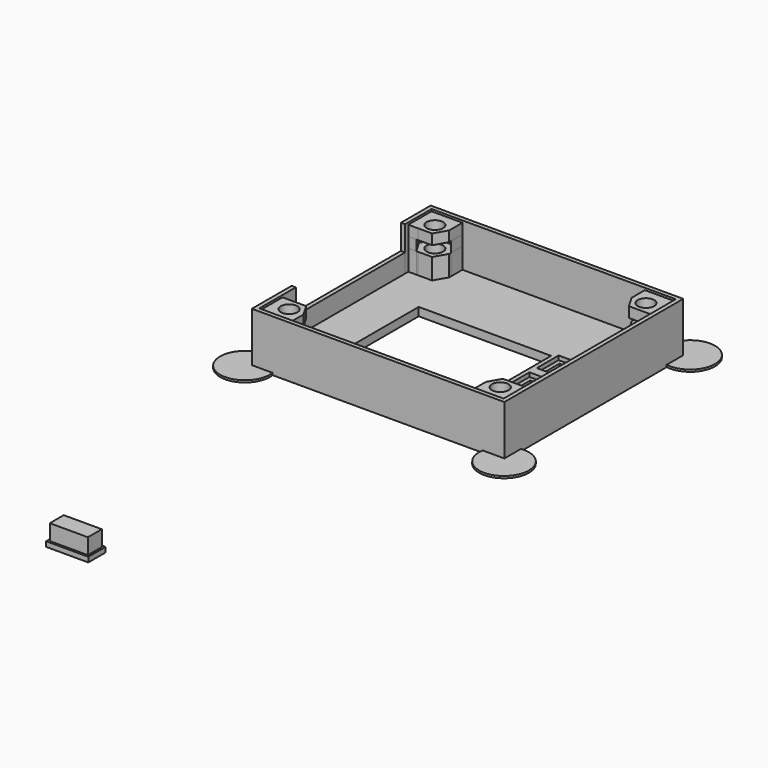
from build123d import *

# Parameters (mm, degrees)
F0_R      = 2
F1_DEPTH  = 7
F2_DEPTH  = 7
F3_DEPTH  = 2.5
F4_START  = 2.5
F1_FACE_R = 2
F4_DEPTH  = 2.5
F0_W      = 32
F0_H      = 23
F0_W_2    = 11.6
F0_H_2    = 6.6
F5_DEPTH  = 2
F0_W_3    = 9.6
F0_H_3    = 4.6
F6_DEPTH  = 1
F7_DEPTH  = 12.5
F0_W_4    = 1
F0_H_4    = 33
F8_DEPTH  = 6.5
F0_W_5    = 10.2
F0_H_5    = 5.2
F0_W_6    = 9.2
F0_H_6    = 4.2
F9_DEPTH  = 1.2
F10_DEPTH = 5
F11_DEPTH = 0.5


with BuildPart() as f1:
    # F0 (on Top) → F1 (new body)
    with BuildSketch(Plane.XY):
        Polygon((56.2425711751, 29.4110085815), (56.2425711751, 36.414245103), (54.3157895307, 36.414245103), (56.0530762776, 33.4181404888), (54.1540001392, 30.1145803152), (50.3434950368, 30.1074484079), (48.7784756274, 32.8064627658), (48.7784756274, 29.4110085815), (52.2425711751, 29.4110085815), align=None)
        Polygon((56.0530762776, 33.4181404888), (54.3157895307, 36.414245103), (53.9690040281, 36.414245103), (50.5049084804, 36.4077615509), (48.7784756274, 33.4045250294), (48.7784756274, 32.8064627658), (50.3434950368, 30.1074484079), (54.1540001392, 30.1145803152), align=None)
        with Locations((52.2425711751, 33.4110085815)):
            Circle(F0_R, mode=Mode.SUBTRACT)
    extrude(amount=F1_DEPTH)


with BuildPart() as f1b:
    # F0 (on Top) → F1, piece 2 (new body)
    with BuildSketch(Plane.XY):
        Polygon((-0.8411283625, 36.4077615509), (-2.7574288249, 36.4077615509), (-2.7574288249, 29.4110085815), (4.7066667228, 29.4110085815), (4.7066667228, 32.8155396842), (3.1540001392, 30.1145803152), (-0.6565049632, 30.1074484079), (-2.5679339274, 33.4038766742), align=None)
        Polygon((-0.4950915196, 36.4077615509), (-0.8411283625, 36.4077615509), (-2.5679339274, 33.4038766742), (-0.6565049632, 30.1074484079), (3.1540001392, 30.1145803152), (4.7066667228, 32.8155396842), (4.7066667228, 33.4174921336), (2.9690040281, 36.414245103), align=None)
        with Locations((1.2425711751, 33.4110085815)):
            Circle(F0_R, mode=Mode.SUBTRACT)
    extrude(amount=F1_DEPTH)


with BuildPart() as f1c:
    # F0 (on Top) → F1, piece 3 (new body)
    with BuildSketch(Plane.XY):
        Polygon((4.7066667228, 81.4110085815), (-2.7574288249, 81.4110085815), (-2.7574288249, 74.40777206), (-0.8306471805, 74.40777206), (-2.5679339274, 77.4038766742), (-0.668857789, 80.7074368479), (3.1416473134, 80.7145687551), (4.7066667228, 78.0155543972), align=None)
        Polygon((4.7066667228, 77.4174921336), (4.7066667228, 78.0155543972), (3.1416473134, 80.7145687551), (-0.668857789, 80.7074368479), (-2.5679339274, 77.4038766742), (-0.8306471805, 74.40777206), (-0.4838616779, 74.40777206), (2.9802338698, 74.4142556121), align=None)
        with Locations((1.2425711751, 77.4110085815)):
            Circle(F0_R, mode=Mode.SUBTRACT)
    extrude(amount=F1_DEPTH)


with BuildPart() as f1d:
    # F0 (on Top) → F1, piece 4 (new body)
    with BuildSketch(Plane.XY):
        Polygon((56.2425711751, 81.4110085815), (48.7784756274, 81.4110085815), (48.7784756274, 78.0064774788), (50.331142211, 80.7074368479), (54.1416473134, 80.7145687551), (56.0530762776, 77.4181404888), (54.3266434245, 74.4149039673), (56.2425711751, 74.4184899011), align=None)
        Polygon((50.331142211, 80.7074368479), (48.7784756274, 78.0064774788), (48.7784756274, 77.4045250294), (50.5161383221, 74.40777206), (53.9802338698, 74.4142556121), (54.3266434245, 74.4149039673), (56.0530762776, 77.4181404888), (54.1416473134, 80.7145687551), align=None)
        with Locations((52.2425711751, 77.4110085815)):
            Circle(F0_R, mode=Mode.SUBTRACT)
    extrude(amount=F1_DEPTH)


with BuildPart() as f2:
    # F0 (on Top) → F2 (new body, through all)
    with BuildSketch(Plane.XY):
        Polygon((56.2425711751, 29.4110085815), (56.2425711751, 36.414245103), (54.3157895307, 36.414245103), (56.0530762776, 33.4181404888), (54.1540001392, 30.1145803152), (50.3434950368, 30.1074484079), (48.7784756274, 32.8064627658), (48.7784756274, 29.4110085815), (52.2425711751, 29.4110085815), align=None)
    extrude(amount=F2_DEPTH)


with BuildPart() as f2b:
    # F0 (on Top) → F2, piece 2 (new body, through all)
    with BuildSketch(Plane.XY):
        Polygon((56.2425711751, 81.4110085815), (48.7784756274, 81.4110085815), (48.7784756274, 78.0064774788), (50.331142211, 80.7074368479), (54.1416473134, 80.7145687551), (56.0530762776, 77.4181404888), (54.3266434245, 74.4149039673), (56.2425711751, 74.4184899011), align=None)
    extrude(amount=F2_DEPTH)


with BuildPart() as f2c:
    # F0 (on Top) → F2, piece 3 (new body, through all)
    with BuildSketch(Plane.XY):
        Polygon((4.7066667228, 81.4110085815), (-2.7574288249, 81.4110085815), (-2.7574288249, 74.40777206), (-0.8306471805, 74.40777206), (-2.5679339274, 77.4038766742), (-0.668857789, 80.7074368479), (3.1416473134, 80.7145687551), (4.7066667228, 78.0155543972), align=None)
    extrude(amount=F2_DEPTH)


with BuildPart() as f2d:
    # F0 (on Top) → F2, piece 4 (new body, through all)
    with BuildSketch(Plane.XY):
        Polygon((-0.8411283625, 36.4077615509), (-2.7574288249, 36.4077615509), (-2.7574288249, 29.4110085815), (4.7066667228, 29.4110085815), (4.7066667228, 32.8155396842), (3.1540001392, 30.1145803152), (-0.6565049632, 30.1074484079), (-2.5679339274, 33.4038766742), align=None)
    extrude(amount=F2_DEPTH)


with BuildPart() as f3:
    # F3 (new): a face of the model
    f3_faces = [f2.part.faces().sort_by_distance(p)[0] for p in [
        (56.1402197979, 32.9126268423, 7),
    ]]
    extrude(f3_faces, amount=F3_DEPTH)

    # F1_face (on face) → F4 (join)
    with BuildSketch(Plane(origin=(52.8230493213, 32.5673462874, 7), x_dir=(1, 0, 0), z_dir=(0, 0, 1)).offset(F4_START)):
        Polygon((3.4195218538, -3.1563377059), (3.4195218538, 3.8468988156), (1.1459547068, 3.8468988156), (-2.3181408409, 3.8404152635), (-4.0445736939, 0.837178742), (-4.0445736939, -3.1563377059), align=None)
        with Locations((-0.5804781462, 0.8436622941)):
            Circle(F1_FACE_R, mode=Mode.SUBTRACT)
    extrude(amount=F4_DEPTH)


with BuildPart() as f3b:
    # F3#2 (new): a face of the model
    f3_2_faces = [f2d.part.faces().sort_by_distance(p)[0] for p in [
        (-1.7007240321, 31.7043432897, 7),
    ]]
    extrude(f3_2_faces, amount=F3_DEPTH)


with BuildPart() as f3c:
    # F3#3 (new): a face of the model
    f3_3_faces = [f2c.part.faces().sort_by_distance(p)[0] for p in [
        (0.9746189489, 81.3086572043, 7),
    ]]
    extrude(f3_3_faces, amount=F3_DEPTH)


with BuildPart() as f3d:
    # F3#4 (new): a face of the model
    f3_4_faces = [f2b.part.faces().sort_by_distance(p)[0] for p in [
        (55.2844158262, 74.5189993465, 7),
    ]]
    extrude(f3_4_faces, amount=F3_DEPTH)


with BuildPart() as f4:
    # F1_face (on face) → F4, piece 2 (new body)
    with BuildSketch(Plane(origin=(52.8230493213, 32.5673462874, 7), x_dir=(1, 0, 0), z_dir=(0, 0, 1)).offset(F4_START)):
        Polygon((-55.5804781462, 3.8404152635), (-55.5804781462, -3.1563377059), (-48.1163825985, -3.1563377059), (-48.1163825985, 0.8501458462), (-49.8540452932, 3.8468988156), (-53.3181408409, 3.8404152635), align=None)
        with Locations((-51.5804781462, 0.8436622941)):
            Circle(F1_FACE_R, mode=Mode.SUBTRACT)
    extrude(amount=F4_DEPTH)


with BuildPart() as f4b:
    # F1_face (on face) → F4, piece 3 (new body)
    with BuildSketch(Plane(origin=(52.8230493213, 32.5673462874, 7), x_dir=(1, 0, 0), z_dir=(0, 0, 1)).offset(F4_START)):
        Polygon((-48.1163825985, 48.8436622941), (-55.5804781462, 48.8436622941), (-55.5804781462, 41.8404257726), (-53.3069109992, 41.8404257726), (-49.8428154515, 41.8469093247), (-48.1163825985, 44.8501458462), align=None)
        with Locations((-51.5804781462, 44.8436622941)):
            Circle(F1_FACE_R, mode=Mode.SUBTRACT)
    extrude(amount=F4_DEPTH)


with BuildPart() as f4c:
    # F1_face (on face) → F4, piece 4 (new body)
    with BuildSketch(Plane(origin=(52.8230493213, 32.5673462874, 7), x_dir=(1, 0, 0), z_dir=(0, 0, 1)).offset(F4_START)):
        Polygon((3.4195218538, 41.8511436137), (3.4195218538, 48.8436622941), (-4.0445736939, 48.8436622941), (-4.0445736939, 44.837178742), (-2.3069109992, 41.8404257726), align=None)
        with Locations((-0.5804781462, 44.8436622941)):
            Circle(F1_FACE_R, mode=Mode.SUBTRACT)
    extrude(amount=F4_DEPTH)


with BuildPart() as f5:
    # F0 (on Top) → F5 (new body)
    with BuildSketch(Plane.XY):
        Polygon((48.7784756274, 81.4110085815), (4.7066667228, 81.4110085815), (4.7066667228, 78.0155543972), (4.7066667228, 77.4174921336), (2.9802338698, 74.4142556121), (-0.4838616779, 74.40777206), (-0.8306471805, 74.40777206), (-2.7574288249, 74.40777206), (-2.7574288249, 73.4110085815), (-2.7574288249, 40.4110085815), (-2.7574288249, 36.4077615509), (-0.8411283625, 36.4077615509), (-0.4950915196, 36.4077615509), (2.9690040281, 36.414245103), (4.7066667228, 33.4174921336), (4.7066667228, 32.8155396842), (4.7066667228, 29.4110085815), (48.7784756274, 29.4110085815), (48.7784756274, 32.8064627658), (48.7784756274, 33.4045250294), (50.5049084804, 36.4077615509), (53.9690040281, 36.414245103), (54.3157895307, 36.414245103), (56.2425711751, 36.414245103), (56.2425711751, 74.4184899011), (54.3266434245, 74.4149039673), (53.9802338698, 74.4142556121), (50.5161383221, 74.40777206), (48.7784756274, 77.4045250294), (48.7784756274, 78.0064774788), align=None)
        with Locations((23.7425711751, 52.9110085815)):
            Rectangle(F0_W, F0_H, mode=Mode.SUBTRACT)
        with Locations((46.5425711751, 43.7110085815)):
            Rectangle(F0_W_2, F0_H_2, mode=Mode.SUBTRACT)
        with Locations((46.5425711751, 53.3110085815)):
            Rectangle(F0_W_2, F0_H_2, mode=Mode.SUBTRACT)
        Polygon((40.7425711751, 65.4110085815), (49.1506871892, 65.4110085815), (52.3425711751, 65.4110085815), (52.3425711751, 58.8110085815), (45.3566280971, 58.8110085815), (40.7425711751, 58.8110085815), align=None, mode=Mode.SUBTRACT)
    extrude(amount=F5_DEPTH)

    # F0 (on Top) → F6 (join)
    with BuildSketch(Plane.XY):
        Polygon((48.575829751, 64.4110085815), (49.1506871892, 65.4110085815), (40.7425711751, 65.4110085815), (40.7425711751, 58.8110085815), (45.3566280971, 58.8110085815), (45.9314855353, 59.8110085815), (41.7425711751, 59.8110085815), (41.7425711751, 64.4110085815), align=None)
        Polygon((52.3425711751, 65.4110085815), (49.1506871892, 65.4110085815), (48.575829751, 64.4110085815), (51.3425711751, 64.4110085815), (51.3425711751, 59.8110085815), (45.9314855353, 59.8110085815), (45.3566280971, 58.8110085815), (52.3425711751, 58.8110085815), align=None)
        with Locations((46.5425711751, 53.3110085815)):
            Rectangle(F0_W_2, F0_H_2)
        with Locations((46.5425711751, 53.3110085815)):
            Rectangle(F0_W_3, F0_H_3, mode=Mode.SUBTRACT)
        with Locations((46.5425711751, 43.7110085815)):
            Rectangle(F0_W_2, F0_H_2)
        with Locations((46.5425711751, 43.7110085815)):
            Rectangle(F0_W_3, F0_H_3, mode=Mode.SUBTRACT)
    extrude(amount=F6_DEPTH)


with BuildPart() as f5b:
    # F0 (on Top) → F5, piece 2 (new body)
    with BuildSketch(Plane.XY):
        with Locations((1.2425711751, 77.4110085815)):
            Circle(F0_R)
    extrude(amount=F5_DEPTH)


with BuildPart() as f5c:
    # F0 (on Top) → F5, piece 3 (new body)
    with BuildSketch(Plane.XY):
        with Locations((52.2425711751, 77.4110085815)):
            Circle(F0_R)
    extrude(amount=F5_DEPTH)


with BuildPart() as f5d:
    # F0 (on Top) → F5, piece 4 (new body)
    with BuildSketch(Plane.XY):
        with Locations((52.2425711751, 33.4110085815)):
            Circle(F0_R)
    extrude(amount=F5_DEPTH)


with BuildPart() as f5e:
    # F0 (on Top) → F5, piece 5 (new body)
    with BuildSketch(Plane.XY):
        with Locations((1.2425711751, 33.4110085815)):
            Circle(F0_R)
    extrude(amount=F5_DEPTH)


with BuildPart() as f7:
    # F0 (on Top) → F7 (new body)
    with BuildSketch(Plane.XY):
        with BuildLine():
            Line((-2.7574288249, 74.40777206), (-2.7574288249, 81.4110085815))
            Line((-2.7574288249, 81.4110085815), (4.7066667228, 81.4110085815))
            Line((4.7066667228, 81.4110085815), (48.7784756274, 81.4110085815))
            Line((48.7784756274, 81.4110085815), (56.2425711751, 81.4110085815))
            Line((56.2425711751, 81.4110085815), (56.2425711751, 74.4184899011))
            Line((56.2425711751, 74.4184899011), (56.2425711751, 36.414245103))
            Line((56.2425711751, 36.414245103), (56.2425711751, 29.4110085815))
            Line((56.2425711751, 29.4110085815), (52.2425711751, 29.4110085815))
            ThreePointArc((52.2425711751, 29.4110085815), (52.0955733964, 28.9164089663), (51.9916138982, 28.4110085815))
            Line((51.9916138982, 28.4110085815), (57.2425711751, 28.4110085815))
            Line((57.2425711751, 28.4110085815), (57.2425711751, 33.4181404888))
            Line((57.2425711751, 33.4181404888), (57.2425711751, 77.4181404888))
            Line((57.2425711751, 77.4181404888), (57.2425711751, 82.4110085815))
            Line((57.2425711751, 82.4110085815), (52.2425711751, 82.4110085815))
            Line((52.2425711751, 82.4110085815), (1.2425711751, 82.4110085815))
            Line((1.2425711751, 82.4110085815), (-3.7574288249, 82.4110085815))
            Line((-3.7574288249, 82.4110085815), (-3.7574288249, 77.4045250294))
            Line((-3.7574288249, 77.4045250294), (-3.7574288249, 73.4110085815))
            Line((-3.7574288249, 73.4110085815), (-2.7574288249, 73.4110085815))
            Line((-2.7574288249, 73.4110085815), (-2.7574288249, 74.40777206))
        make_face()
        with BuildLine():
            Line((-2.7574288249, 36.4077615509), (-2.7574288249, 40.4110085815))
            Line((-2.7574288249, 40.4110085815), (-3.7574288249, 40.4110085815))
            Line((-3.7574288249, 40.4110085815), (-3.7574288249, 33.4038766742))
            Line((-3.7574288249, 33.4038766742), (-3.7574288249, 28.4110085815))
            Line((-3.7574288249, 28.4110085815), (1.2425711751, 28.4110085815))
            Line((1.2425711751, 28.4110085815), (51.9916138982, 28.4110085815))
            ThreePointArc((51.9916138982, 28.4110085815), (52.0955733964, 28.9164089663), (52.2425711751, 29.4110085815))
            Line((52.2425711751, 29.4110085815), (48.7784756274, 29.4110085815))
            Line((48.7784756274, 29.4110085815), (4.7066667228, 29.4110085815))
            Line((4.7066667228, 29.4110085815), (-2.7574288249, 29.4110085815))
            Line((-2.7574288249, 29.4110085815), (-2.7574288249, 36.4077615509))
        make_face()
    extrude(amount=F7_DEPTH)

    # F0 (on Top) → F11 (join)
    with BuildSketch(Plane.XY):
        with BuildLine():
            Line((-3.7574288249, 28.4110085815), (-3.7574288249, 33.4038766742))
            ThreePointArc((-3.7574288249, 33.4038766742), (-8.9237187174, 23.2302020618), (1.2425711751, 28.4110085815))
            Line((1.2425711751, 28.4110085815), (-3.7574288249, 28.4110085815))
        make_face()
        with BuildLine():
            ThreePointArc((1.2425711751, 82.4110085815), (-8.9316812756, 87.5720808603), (-3.7574288249, 77.4045250294))
            Line((-3.7574288249, 77.4045250294), (-3.7574288249, 82.4110085815))
            Line((-3.7574288249, 82.4110085815), (1.2425711751, 82.4110085815))
        make_face()
        with BuildLine():
            ThreePointArc((57.2425711751, 77.4181404888), (62.4088610676, 87.5918151013), (52.2425711751, 82.4110085815))
            Line((52.2425711751, 82.4110085815), (57.2425711751, 82.4110085815))
            Line((57.2425711751, 82.4110085815), (57.2425711751, 77.4181404888))
        make_face()
        with BuildLine():
            Line((57.2425711751, 28.4110085815), (51.9916138982, 28.4110085815))
            ThreePointArc((51.9916138982, 28.4110085815), (62.0557427442, 23.1136946779), (57.2425711751, 33.4181404888))
            Line((57.2425711751, 33.4181404888), (57.2425711751, 28.4110085815))
        make_face()
    extrude(amount=F11_DEPTH)


with BuildPart() as f8:
    # F0 (on Top) → F8 (new body)
    with BuildSketch(Plane.XY):
        with Locations((-3.2574288249, 56.9110085815)):
            Rectangle(F0_W_4, F0_H_4)
    extrude(amount=F8_DEPTH)


with BuildPart() as f9:
    # F0 (on Top) → F9 (new body)
    with BuildSketch(Plane.XY):
        with Locations((16.7951593995, -50.4477024078)):
            Rectangle(F0_W_5, F0_H_5)
        with Locations((16.7951593995, -50.4477024078)):
            Rectangle(F0_W_6, F0_H_6, mode=Mode.SUBTRACT)
    extrude(amount=F9_DEPTH)

    # F0 (on Top) → F10 (join)
    with BuildSketch(Plane.XY):
        with Locations((16.7951593995, -50.4477024078)):
            Rectangle(F0_W_6, F0_H_6)
    extrude(amount=F10_DEPTH)


solid = Compound([f1.part, f1b.part, f1c.part, f1d.part, f2.part, f2b.part, f2c.part, f2d.part, f3.part, f3b.part, f3c.part, f3d.part, f4.part, f4b.part, f4c.part, f5.part, f5b.part, f5c.part, f5d.part, f5e.part, f7.part, f8.part, f9.part])
